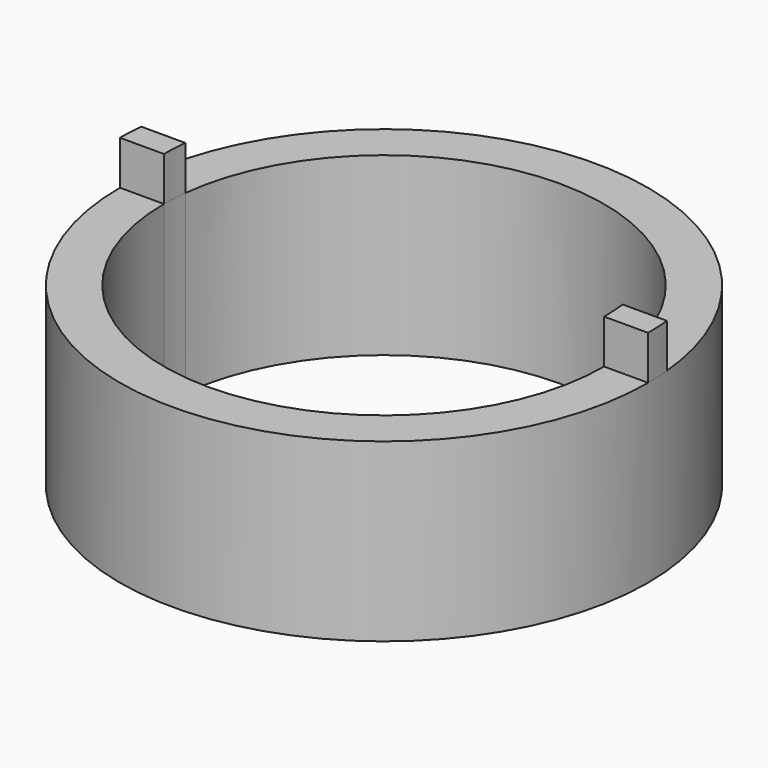
from build123d import *

# Parameters (mm, degrees)
F1_DEPTH = 6.35
F2_DEPTH = 25.4


with BuildPart() as f1:
    # F0 (on Top) → F1 (new body)
    with BuildSketch(Plane.XY):
        with BuildLine():
            Line((31.75, 0), (38.1, 0))
            ThreePointArc((38.1, 0), (38.0570298857, 1.8089986952), (37.9282164683, 3.6139169242))
            Line((37.9282164683, 3.6139169242), (31.5436539492, 3.6139169242))
            ThreePointArc((31.5436539492, 3.6139169242), (31.6983715109, 1.8099015324), (31.75, 0))
        make_face()
    extrude(amount=F1_DEPTH)


with BuildPart() as f1b:
    # F0 (on Top) → F1, piece 2 (new body)
    with BuildSketch(Plane.XY):
        with BuildLine():
            ThreePointArc((-37.9282164683, 3.6139169242), (-38.0570298857, 1.8089986952), (-38.1, 0))
            Line((-38.1, 0), (-31.75, 0))
            ThreePointArc((-31.75, 0), (-31.6983715109, 1.8099015324), (-31.5436539492, 3.6139169242))
            Line((-31.5436539492, 3.6139169242), (-37.9282164683, 3.6139169242))
        make_face()
    extrude(amount=F1_DEPTH)


with BuildPart() as f2:
    # F0 (on Top) → F2 (new body)
    with BuildSketch(Plane.XY):
        with BuildLine():
            Line((31.75, 0), (38.1, 0))
            ThreePointArc((38.1, 0), (38.0570298857, 1.8089986952), (37.9282164683, 3.6139169242))
            Line((37.9282164683, 3.6139169242), (31.5436539492, 3.6139169242))
            ThreePointArc((31.5436539492, 3.6139169242), (31.6983715109, 1.8099015324), (31.75, 0))
        make_face()
        with BuildLine():
            ThreePointArc((-38.1, 0), (0, -38.1), (38.1, 0))
            Line((38.1, 0), (31.75, 0))
            ThreePointArc((31.75, 0), (0, -31.75), (-31.75, 0))
            Line((-31.75, 0), (-38.1, 0))
        make_face()
        with BuildLine():
            Line((31.5436539492, 3.6139169242), (37.9282164683, 3.6139169242))
            ThreePointArc((37.9282164683, 3.6139169242), (0, 38.1), (-37.9282164683, 3.6139169242))
            Line((-37.9282164683, 3.6139169242), (-31.5436539492, 3.6139169242))
            ThreePointArc((-31.5436539492, 3.6139169242), (0, 31.75), (31.5436539492, 3.6139169242))
        make_face()
        with BuildLine():
            ThreePointArc((-37.9282164683, 3.6139169242), (-38.0570298857, 1.8089986952), (-38.1, 0))
            Line((-38.1, 0), (-31.75, 0))
            ThreePointArc((-31.75, 0), (-31.6983715109, 1.8099015324), (-31.5436539492, 3.6139169242))
            Line((-31.5436539492, 3.6139169242), (-37.9282164683, 3.6139169242))
        make_face()
    extrude(amount=-F2_DEPTH)


solid = Compound([f1.part, f1b.part, f2.part])
